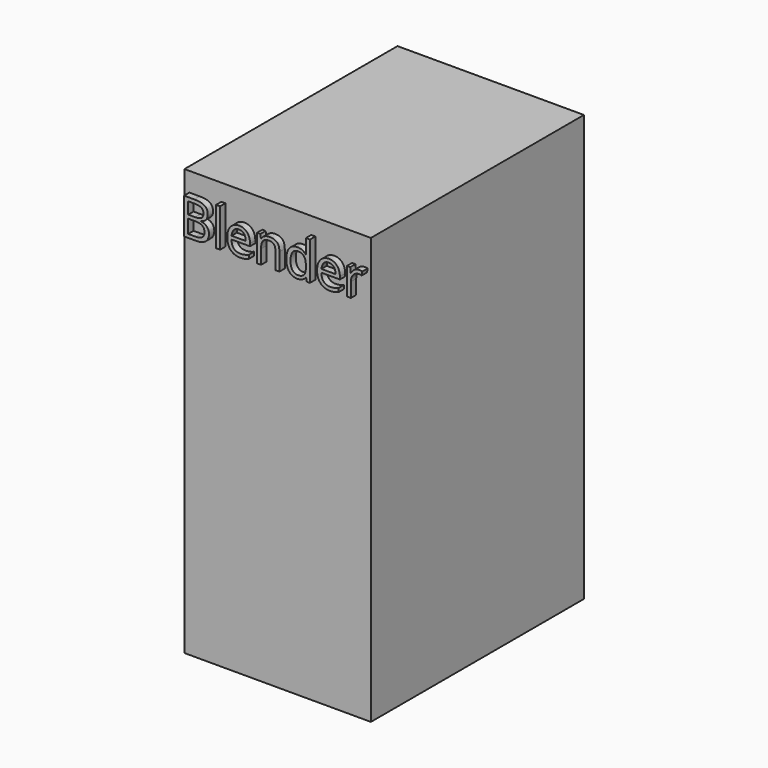
from build123d import *

# Parameters (mm, degrees)
F0_W         = 177.8
F0_H         = 406.4
F1_DEPTH     = 254
F2_TEXT_SIZE = 47.942700653
F3_DEPTH     = 6.35


# Not quite as in the source:
# - Text() gives the source's letters only with a copy of the font that has no kerning and outlines rounded to 1/6400 em; it was checked with that copy


with BuildPart() as f1:
    # F0 (on Front) → F1 (new body)
    with BuildSketch(Plane.XZ):
        with Locations((88.9, 203.2)):
            Rectangle(F0_W, F0_H)
    extrude(amount=F1_DEPTH)

    # F2 (on face) → F3 (join)
    with BuildSketch(Plane.XZ.offset(254)):
        with Locations((0, 353.9583398496)):
            Text('Blender', F2_TEXT_SIZE, font='Open Sans', text_align=(TextAlign.LEFT, TextAlign.BOTTOM))
    extrude(amount=F3_DEPTH)


solid = f1.part
